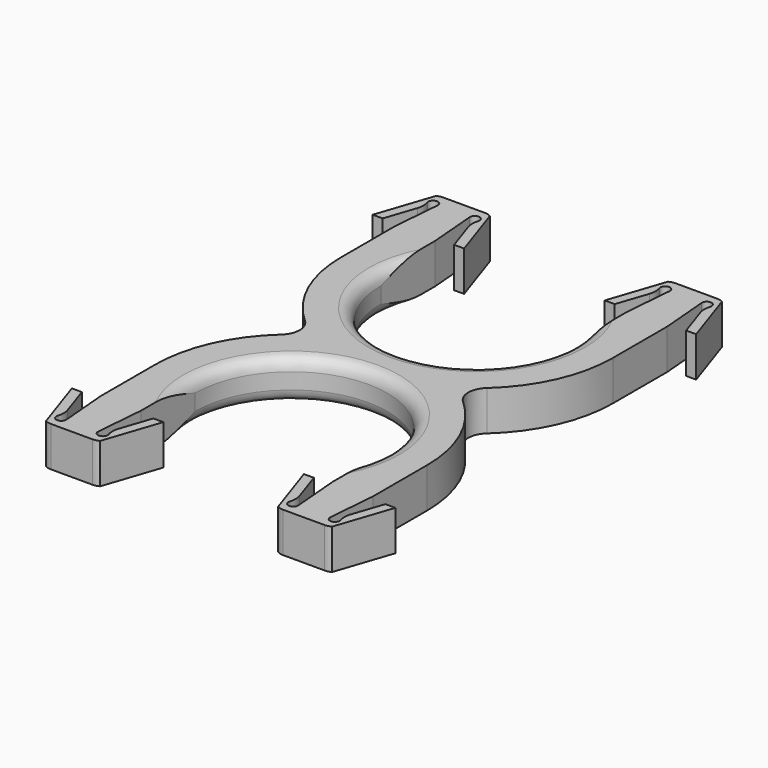
from build123d import *

# Parameters (mm, degrees)
F1_DEPTH    = 10
F2_T2_ANGLE = 240.9746670828
F2_T4_ANGLE = 240.9746670828
F2_T6_ANGLE = 240.9746670828
F2_T8_ANGLE = 240.9746670828


# Not quite as in the source:
# - a fillet or chamfer that OpenCascade refuses, or shapes differently, is made with other operations: its cross-section is extruded or revolved along the edge and cut away or added


with BuildPart() as f1:
    # F0 (on Top) → F1 (new body)
    with BuildSketch(Plane.XY):
        with BuildLine():
            ThreePointArc((6.3393482774, 11.7357549763), (6.1040734685, 10.1783374237), (6.3649625736, 8.6250053459))
            Line((6.3649625736, 8.6250053459), (8.9305315263, 1))
            Line((8.9305315263, 1), (11.4305315263, 1))
            Line((11.4305315263, 1), (6.7557454084, 14.8937092698))
            ThreePointArc((6.7557454084, 14.8937092698), (6.001778287, 15.1965058009), (5.1958549099, 15.2996545758))
            Line((5.1958549099, 15.2996545758), (0, 15.2996545758))
            Line((0, 15.2996545758), (-5.1958549099, 15.2996545758))
            ThreePointArc((-5.1958549099, 15.2996545758), (-6.001778287, 15.1965058009), (-6.7557454084, 14.8937092698))
            Line((-6.7557454084, 14.8937092698), (-11.4305315263, 1))
            Line((-11.4305315263, 1), (-8.9305315263, 1))
            Line((-8.9305315263, 1), (-6.3649625736, 8.6250053459))
            ThreePointArc((-6.3649625736, 8.6250053459), (-6.1040734685, 10.1783374237), (-6.3393482774, 11.7357549763))
            ThreePointArc((-6.3393482774, 11.7357549763), (-5.3305463755, 13.2920715369), (-4, 12))
            Line((-4, 12), (-5, 0))
            Line((-5, 0), (-5, -17))
            ThreePointArc((-5, -17), (-2.0559445405, -30.8393753001), (6.2663710998, -42.2820512821))
            ThreePointArc((6.2663710998, -42.2820512821), (7.9231903792, -46), (6.2663710998, -49.7179487179))
            ThreePointArc((6.2663710998, -49.7179487179), (-2.0559445405, -61.1606246999), (-5, -75))
            Line((-5, -75), (-5, -92))
            Line((-5, -92), (-4, -104))
            ThreePointArc((-4, -104), (-5.3305463755, -105.2920715369), (-6.3393482774, -103.7357549763))
            ThreePointArc((-6.3393482774, -103.7357549763), (-6.1040734685, -102.1783374237), (-6.3649625736, -100.6250053459))
            Line((-6.3649625736, -100.6250053459), (-8.9305315263, -93))
            Line((-8.9305315263, -93), (-11.4305315263, -93))
            Line((-11.4305315263, -93), (-6.7557454084, -106.8937092698))
            ThreePointArc((-6.7557454084, -106.8937092698), (-6.001778287, -107.1965058009), (-5.1958549099, -107.2996545758))
            Line((-5.1958549099, -107.2996545758), (0, -107.2996545758))
            Line((0, -107.2996545758), (5.1958549099, -107.2996545758))
            ThreePointArc((5.1958549099, -107.2996545758), (6.001778287, -107.1965058009), (6.7557454084, -106.8937092698))
            Line((6.7557454084, -106.8937092698), (11.4305315263, -93))
            Line((11.4305315263, -93), (8.9305315263, -93))
            Line((8.9305315263, -93), (6.3649625736, -100.6250053459))
            ThreePointArc((6.3649625736, -100.6250053459), (6.1040734685, -102.1783374237), (6.3393482774, -103.7357549763))
            ThreePointArc((6.3393482774, -103.7357549763), (5.3305463755, -105.2920715369), (4, -104))
            Line((4, -104), (5, -92))
            Line((5, -92), (5, -75))
            ThreePointArc((5, -75), (29, -51), (53, -75))
            Line((53, -75), (53, -92))
            Line((53, -92), (54, -104))
            ThreePointArc((54, -104), (52.6694536245, -105.2920715369), (51.6606517226, -103.7357549763))
            ThreePointArc((51.6606517226, -103.7357549763), (51.8959265315, -102.1783374237), (51.6350374264, -100.6250053459))
            Line((51.6350374264, -100.6250053459), (49.0694684737, -93))
            Line((49.0694684737, -93), (46.5694684737, -93))
            Line((46.5694684737, -93), (51.2442545916, -106.8937092698))
            ThreePointArc((51.2442545916, -106.8937092698), (51.998221713, -107.1965058009), (52.8041450901, -107.2996545758))
            Line((52.8041450901, -107.2996545758), (58, -107.2996545758))
            Line((58, -107.2996545758), (63.1958549099, -107.2996545758))
            ThreePointArc((63.1958549099, -107.2996545758), (64.001778287, -107.1965058009), (64.7557454084, -106.8937092698))
            Line((64.7557454084, -106.8937092698), (69.4305315263, -93))
            Line((69.4305315263, -93), (66.9305315263, -93))
            Line((66.9305315263, -93), (64.3649625736, -100.6250053459))
            ThreePointArc((64.3649625736, -100.6250053459), (64.1040734685, -102.1783374237), (64.3393482774, -103.7357549763))
            ThreePointArc((64.3393482774, -103.7357549763), (63.3305463755, -105.2920715369), (62, -104))
            Line((62, -104), (63, -92))
            Line((63, -92), (63, -75))
            ThreePointArc((63, -75), (60.0559445405, -61.1606246999), (51.7336289002, -49.7179487179))
            ThreePointArc((51.7336289002, -49.7179487179), (50.0768096208, -46), (51.7336289002, -42.2820512821))
            ThreePointArc((51.7336289002, -42.2820512821), (60.0559445405, -30.8393753001), (63, -17))
            Line((63, -17), (63, 0))
            Line((63, 0), (62, 12))
            ThreePointArc((62, 12), (63.3305463755, 13.2920715369), (64.3393482774, 11.7357549763))
            ThreePointArc((64.3393482774, 11.7357549763), (64.1040734685, 10.1783374237), (64.3649625736, 8.6250053459))
            Line((64.3649625736, 8.6250053459), (66.9305315263, 1))
            Line((66.9305315263, 1), (69.4305315263, 1))
            Line((69.4305315263, 1), (64.7557454084, 14.8937092698))
            ThreePointArc((64.7557454084, 14.8937092698), (64.001778287, 15.1965058009), (63.1958549099, 15.2996545758))
            Line((63.1958549099, 15.2996545758), (58, 15.2996545758))
            Line((58, 15.2996545758), (52.8041450901, 15.2996545758))
            ThreePointArc((52.8041450901, 15.2996545758), (51.998221713, 15.1965058009), (51.2442545916, 14.8937092698))
            Line((51.2442545916, 14.8937092698), (46.5694684737, 1))
            Line((46.5694684737, 1), (49.0694684737, 1))
            Line((49.0694684737, 1), (51.6350374264, 8.6250053459))
            ThreePointArc((51.6350374264, 8.6250053459), (51.8959265315, 10.1783374237), (51.6606517226, 11.7357549763))
            ThreePointArc((51.6606517226, 11.7357549763), (52.6694536245, 13.2920715369), (54, 12))
            Line((54, 12), (53, 0))
            Line((53, 0), (53, -17))
            ThreePointArc((53, -17), (29, -41), (5, -17))
            Line((5, -17), (5, 0))
            Line((5, 0), (4, 12))
            ThreePointArc((4, 12), (5.3305463755, 13.2920715369), (6.3393482774, 11.7357549763))
        make_face()
    extrude(amount=F1_DEPTH)

    # F2: fillet of radius 3 on 4 edges, made by hand

    # F2_s1 → F2_t2 (revolve, cut)
    with BuildSketch(Plane(origin=(14.8970987107, -25.3030447424, 0), x_dir=(0, 0, 1), z_dir=(-0.507347869, 0.8617413416, 0))):
        with BuildLine():
            ThreePointArc((10, 43.3655851338), (9.1213203436, 41.2442647902), (7, 40.3655851338))
            Line((7, 40.3655851338), (10, 40.3655851338))
            Line((10, 40.3655851338), (10, 43.3655851338))
        make_face()
    revolve(axis=Axis((29, -17, 10), (0, 0, -1)), revolution_arc=F2_T2_ANGLE, mode=Mode.SUBTRACT)

    # F2_s3 → F2_t4 (revolve, cut)
    with BuildSketch(Plane(origin=(14.8970987107, -25.3030447424, 0), x_dir=(0, 0, 1), z_dir=(-0.507347869, 0.8617413416, 0))):
        with BuildLine():
            ThreePointArc((3, 40.3655851338), (0.8786796564, 41.2442647902), (0, 43.3655851338))
            Line((0, 43.3655851338), (0, 40.3655851338))
            Line((0, 40.3655851338), (3, 40.3655851338))
        make_face()
    revolve(axis=Axis((29, -17, 0), (0, 0, -1)), revolution_arc=F2_T4_ANGLE, mode=Mode.SUBTRACT)

    # F2_s5 → F2_t6 (revolve, cut)
    with BuildSketch(Plane(origin=(40.2548514411, -68.3737368527, 0), x_dir=(0, 0, 1), z_dir=(0.507347869, -0.8617413416, 0))):
        with BuildLine():
            ThreePointArc((10, 40.0605912676), (9.1213203436, 37.939270924), (7, 37.0605912676))
            Line((7, 37.0605912676), (10, 37.0605912676))
            Line((10, 37.0605912676), (10, 40.0605912676))
        make_face()
    revolve(axis=Axis((29, -75, 10), (0, 0, -1)), revolution_arc=F2_T6_ANGLE, mode=Mode.SUBTRACT)

    # F2_s7 → F2_t8 (revolve, cut)
    with BuildSketch(Plane(origin=(40.2548514411, -68.3737368527, 0), x_dir=(0, 0, 1), z_dir=(0.507347869, -0.8617413416, 0))):
        with BuildLine():
            ThreePointArc((3, 37.0605912676), (0.8786796564, 37.939270924), (0, 40.0605912676))
            Line((0, 40.0605912676), (0, 37.0605912676))
            Line((0, 37.0605912676), (3, 37.0605912676))
        make_face()
    revolve(axis=Axis((29, -75, 0), (0, 0, -1)), revolution_arc=F2_T8_ANGLE, mode=Mode.SUBTRACT)


solid = f1.part
